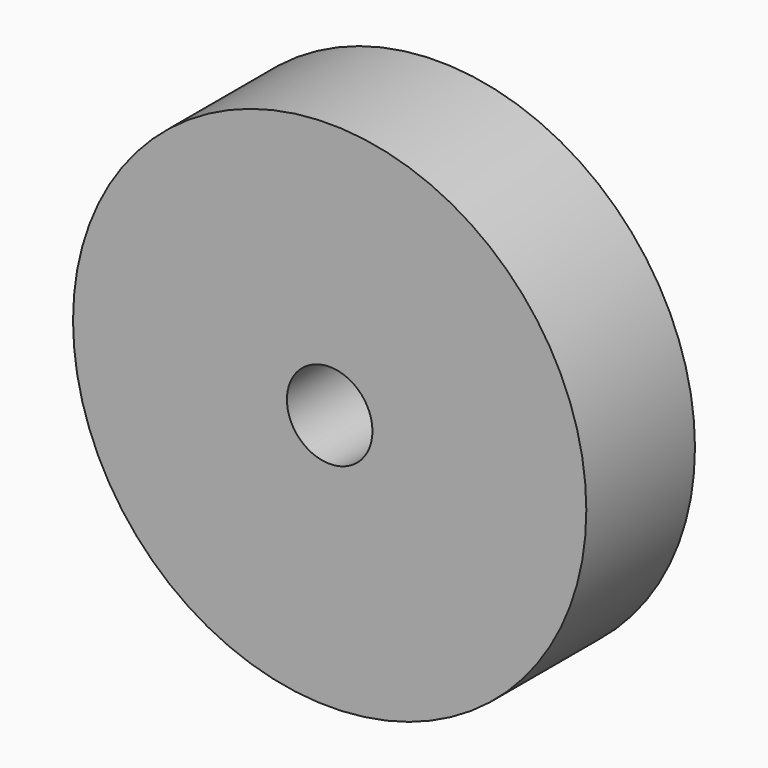
from build123d import *

# Parameters (mm, degrees)
F0_R     = 6
F0_R_2   = 1
F1_DEPTH = 3.175


# Not quite as in the source:
# - a length typed as a fraction of an inch, garbled in the dataset ("3 / 203.2 mm" for 3/8 in), is restored


with BuildPart() as f1:
    # F0 (on Front) → F1 (new body)
    with BuildSketch(Plane.XZ):
        with Locations((-37.8119088709, 24.9558594078)):
            Circle(F0_R)
        with Locations((-37.8119088709, 24.9558594078)):
            Circle(F0_R_2, mode=Mode.SUBTRACT)
    extrude(amount=F1_DEPTH)


solid = f1.part
